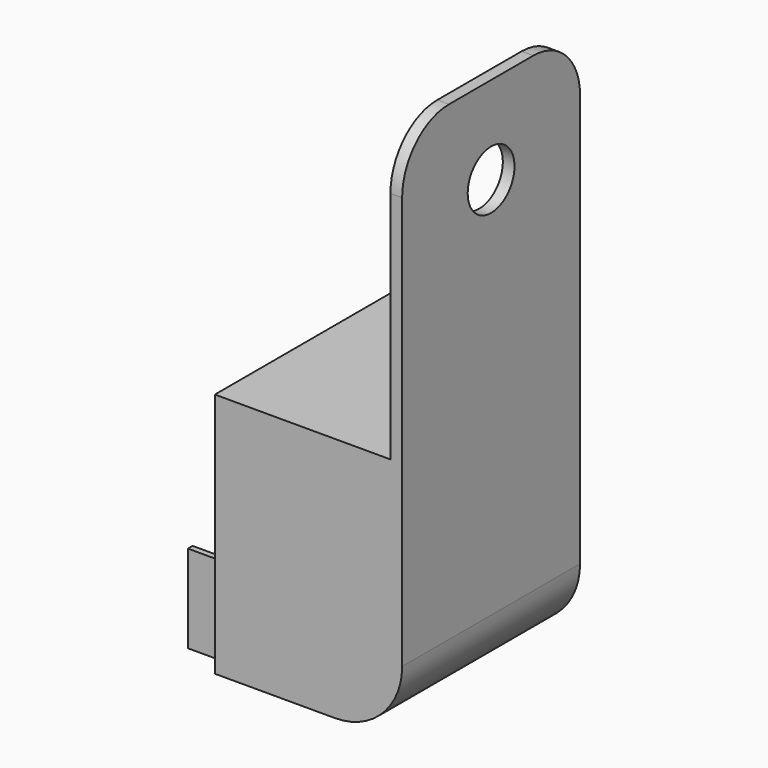
from build123d import *

# Parameters (mm, degrees)
F1_DEPTH  = 38
F3_D      = 12
F5_DEPTH  = 2
F6_R      = 10
F8_D      = 10
F10_DEPTH = 2
F12_DEPTH = 2
F14_W     = 30
F14_H     = 36
F15_DEPTH = 2
F16_W     = 1
F16_H     = 15
F17_DEPTH = 5


# Not quite as in the source:
# - a feature names something its author has since deleted; it is built from what else it names


with BuildPart() as f1:
    # F0 (on Front) → F1 (new body)
    with BuildSketch(Plane.XZ):
        with BuildLine():
            Line((20, 0), (0, 0))
            Line((0, 0), (0, -2))
            Line((0, -2), (20.5, -2))
            ThreePointArc((20.5, -2), (28.6317279836, 1.3682720164), (32, 9.5))
            Line((32, 9.5), (32, 90))
            Line((32, 90), (30, 90))
            Line((30, 90), (30, 10))
            ThreePointArc((30, 10), (27.0710678119, 2.9289321881), (20, 0))
        make_face()
    extrude(amount=F1_DEPTH)

    # F3 (through all)
    with Locations(Plane.XY):
        with Locations((5, -19)):
            Hole(F3_D / 2)

    # F4 (on face) → F5 (join)
    with BuildSketch(Plane(origin=(0, 0, -2), x_dir=(1, 0, 0), z_dir=(0, 0, -1))):
        with BuildLine():
            ThreePointArc((1, 29.246950766), (6.1242290384, 29.9423996029), (11, 28.2195444573))
            ThreePointArc((11, 28.2195444573), (11.8405728739, 27.8759539642), (12.6811457479, 28.2195444573))
            ThreePointArc((12.6811457479, 28.2195444573), (7.117566826, 30.811685347), (1, 30.313708499))
            ThreePointArc((1, 30.313708499), (0.5841901068, 29.7803296325), (1, 29.246950766))
        make_face()
        with BuildLine():
            ThreePointArc((11, 9.7804555427), (6.1242290384, 8.0576003971), (1, 8.753049234))
            ThreePointArc((1, 8.753049234), (0.5841901068, 8.2196703675), (1, 7.686291501))
            ThreePointArc((1, 7.686291501), (7.117566826, 7.188314653), (12.6811457479, 9.7804555427))
            ThreePointArc((12.6811457479, 9.7804555427), (11.8405728739, 10.1240460358), (11, 9.7804555427))
        make_face()
    extrude(amount=F5_DEPTH)

    # F6
    f6_edges = [f1.edges().sort_by_distance(p)[0] for p in [
        (31, -38, 90),
        (31, 0, 90),
    ]]
    fillet(f6_edges, radius=F6_R)

    # F8 (through all)
    with Locations(Plane.YZ.offset(32)):
        with Locations((-19, 75)):
            Hole(F8_D / 2)


with BuildPart() as f10:
    # F9 (on face) → F10 (new body)
    with BuildSketch(Plane.XZ.offset(38)):
        with BuildLine():
            Line((0, 40), (0, 0))
            Line((0, 0), (20, 0))
            ThreePointArc((20, 0), (27.0710678119, 2.9289321881), (30, 10))
            Line((30, 10), (30, 40))
            Line((30, 40), (0, 40))
        make_face()
    extrude(amount=-F10_DEPTH)


with BuildPart() as f12:
    # F11 (on face) → F12 (new body)
    with BuildSketch(Plane(origin=(0, 0, 0), x_dir=(-1, 0, 0), z_dir=(0, 1, 0))):
        with BuildLine():
            Line((-20, 0), (0, 0))
            Line((0, 0), (0, 40))
            Line((0, 40), (-30, 40))
            Line((-30, 40), (-30, 10))
            ThreePointArc((-30, 10), (-27.0710678119, 2.9289321881), (-20, 0))
        make_face()
    extrude(amount=-F12_DEPTH)


with BuildPart() as f1_1:
    add(f1.part)

    # F13: union F10, F12
    add(f10.part)
    add(f12.part)

    # F14 (on face) → F15 (join)
    with BuildSketch(Plane.XY.offset(40)):
        with Locations((15, -20)):
            Rectangle(F14_W, F14_H)
    extrude(amount=-F15_DEPTH)

    # F16 (on face) → F17 (join)
    with BuildSketch(Plane(origin=(0, 0, 0), x_dir=(0, -1, 0), z_dir=(-1, 0, 0))):
        with Locations((37, 7.5)):
            Rectangle(F16_W, F16_H)
    extrude(amount=F17_DEPTH)


solid = f1_1.part
